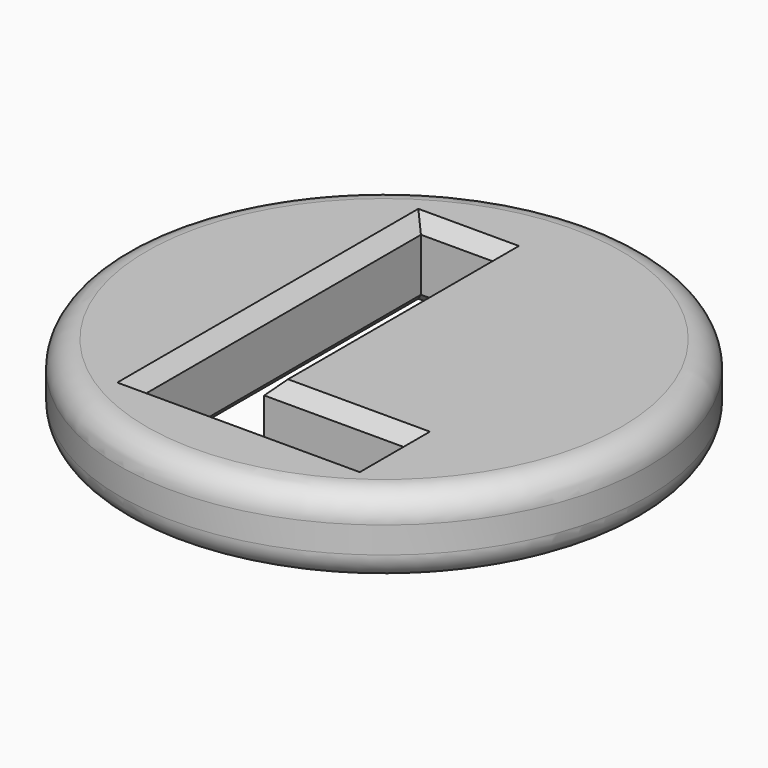
from build123d import *

# Parameters (mm, degrees)
F0_R         = 10
F1_DEPTH     = 3
F2_R         = 1
F3_TEXT_SIZE = 18.56881556
F4_DEPTH     = 6
F5_SIZE      = 0.5


# Not quite as in the source:
# - Text() gives the source's letters only with a copy of the font that has no kerning and outlines rounded to 1/6400 em; it was checked with that copy


with BuildPart() as f1:
    # F0 (on Top) → F1 (new body)
    with BuildSketch(Plane.XY):
        Circle(F0_R)
    extrude(amount=F1_DEPTH)

    # F2
    f2_edges = [f1.edges().sort_by_distance(p)[0] for p in [
        (-10, 0, 3),
        (-10, 0, 0),
    ]]
    fillet(f2_edges, radius=F2_R)

    # F3 (on face) → F4 (cut)
    with BuildSketch(Plane.XY.offset(3)):
        with Locations((-5.5901859887, -6.6084894352)):
            Text('L', F3_TEXT_SIZE, font='Open Sans', font_style=FontStyle.BOLD, text_align=(TextAlign.LEFT, TextAlign.BOTTOM))
    extrude(amount=-F4_DEPTH, mode=Mode.SUBTRACT)

    # F5
    f5_edges = [f1.edges().sort_by_distance(p)[0] for p in [
        (-3.921894, 0.019707, 3),
        (-1.110459, 1.180258, 3),
        (1.577667, -4.287387, 3),
        (-2.516177, 6.647904, 3),
        (0.17195, -6.608489, 3),
        (4.265793, -5.447938, 3),
        (-1.110459, 1.180258, 0),
        (-2.516177, 6.647904, 0),
        (-9, 0, 0),
        (-3.921894, 0.019707, 0),
        (0.17195, -6.608489, 0),
        (4.265793, -5.447938, 0),
        (1.577667, -4.287387, 0),
    ]]
    chamfer(f5_edges, length=F5_SIZE)


solid = f1.part
